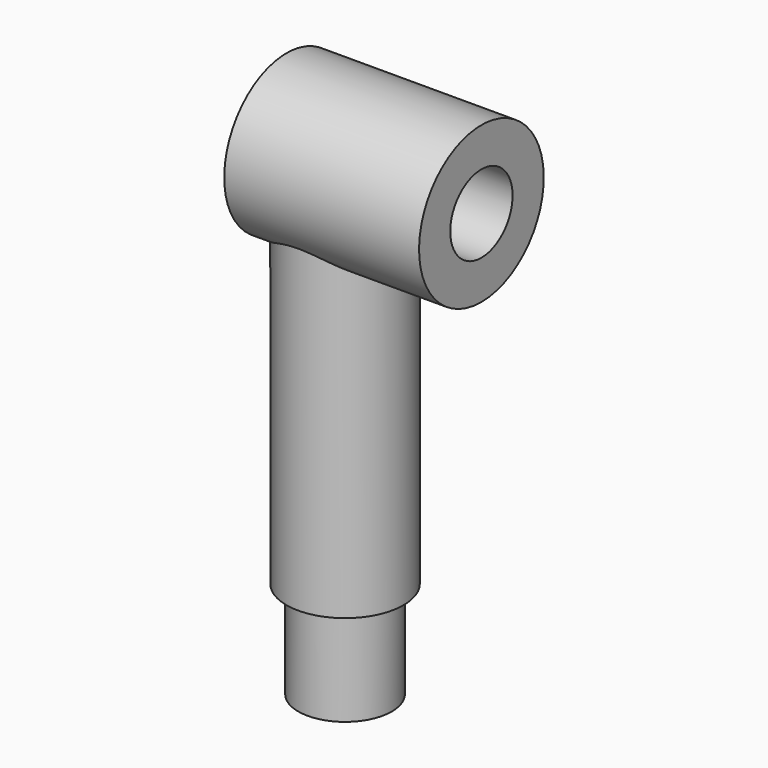
from build123d import *

# Parameters (mm, degrees)
F0_W     = 1.5
F0_H     = 10
F3_DEPTH = 1
F4_R     = 1.5
F4_R_2   = 1.2
F5_DEPTH = 2.5
F4_R_3   = 1
F6_DEPTH = 4


with BuildPart() as f1:
    # F0 (on Front) → F1 (revolve)
    with BuildSketch(Plane.XZ):
        Polygon((-3.5, 0), (0, 0), (0, 1), (-5, 1), (-5, 0), align=None)
    revolve(axis=Axis((-0.3362700678, 0, 2), (1, 0, 0)))



with BuildPart() as f2:
    # F0 (on Front) → F2 (revolve)
    with BuildSketch(Plane.XZ):
        with Locations((-4.25, -5)):
            Rectangle(F0_W, F0_H)
    revolve(axis=Axis((-3.5, 0, -5), (0, 0, -1)))


with BuildPart() as f1_1:
    add(f1.part)
    # F3 (add): a face of the model
    f3_faces = [f2.part.faces().sort_by_distance(p)[0] for p in [
        (-3.5, 0, 0),
    ]]

    add(f2.part)  # F3 merges F2
    extrude(f3_faces, amount=F3_DEPTH)

    # F4 (on face) → F5 (cut)
    with BuildSketch(Plane(origin=(0, 0, -10), x_dir=(1, 0, 0), z_dir=(0, 0, -1))):
        with Locations((-3.5, 0)):
            Circle(F4_R)
        with Locations((-3.5, 0)):
            Circle(F4_R_2, mode=Mode.SUBTRACT)
    extrude(amount=-F5_DEPTH, mode=Mode.SUBTRACT)

    # F4 (on face) → F6 (cut)
    with BuildSketch(Plane(origin=(0, 0, -10), x_dir=(1, 0, 0), z_dir=(0, 0, -1))):
        with Locations((-3.5, 0)):
            Circle(F4_R_3)
    extrude(amount=-F6_DEPTH, mode=Mode.SUBTRACT)


solid = f1_1.part
